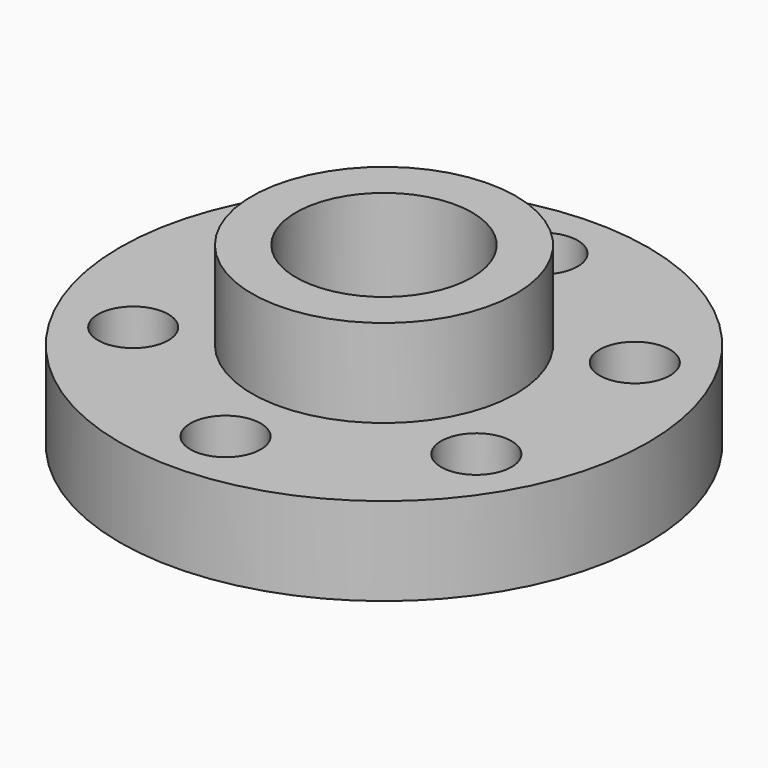
from build123d import *

# Parameters (mm, degrees)
F0_R            = 30
F0_R_2          = 10
F1_DEPTH        = 10
F2_R            = 15
F2_R_2          = 10
F3_DEPTH        = 10
F4_R            = 4
F5_DEPTH        = 10.001
F5_COPIES_COUNT = 6


# Not quite as in the source:
# - a pattern or mirror of a feature is missing from the dataset's text; its kind, count and spacing are read off the source's solid


with BuildPart() as f1:
    # F0 (on Top) → F1 (new body)
    with BuildSketch(Plane.XY):
        Circle(F0_R)
        Circle(F0_R_2, mode=Mode.SUBTRACT)
    extrude(amount=F1_DEPTH)

    # F2 (on face) → F3 (join)
    with BuildSketch(Plane.XY.offset(10)):
        Circle(F2_R)
        Circle(F2_R_2, mode=Mode.SUBTRACT)
    extrude(amount=F3_DEPTH)

    # F4 (on face) → F5 (cut, through all)
    with BuildSketch(Plane.XY.offset(10)):
        with Locations((0, 22.5)):
            Circle(F4_R)
    f5 = extrude(amount=-F5_DEPTH, mode=Mode.SUBTRACT)

    # F5_copies: F5 ×6 about axis
    f5_copies_axis = Axis((0, 0, 0), (0, 0, 1))
    for i in range(1, F5_COPIES_COUNT):
        add(f5.rotate(f5_copies_axis, i * 360 / F5_COPIES_COUNT), mode=Mode.SUBTRACT)


solid = f1.part
